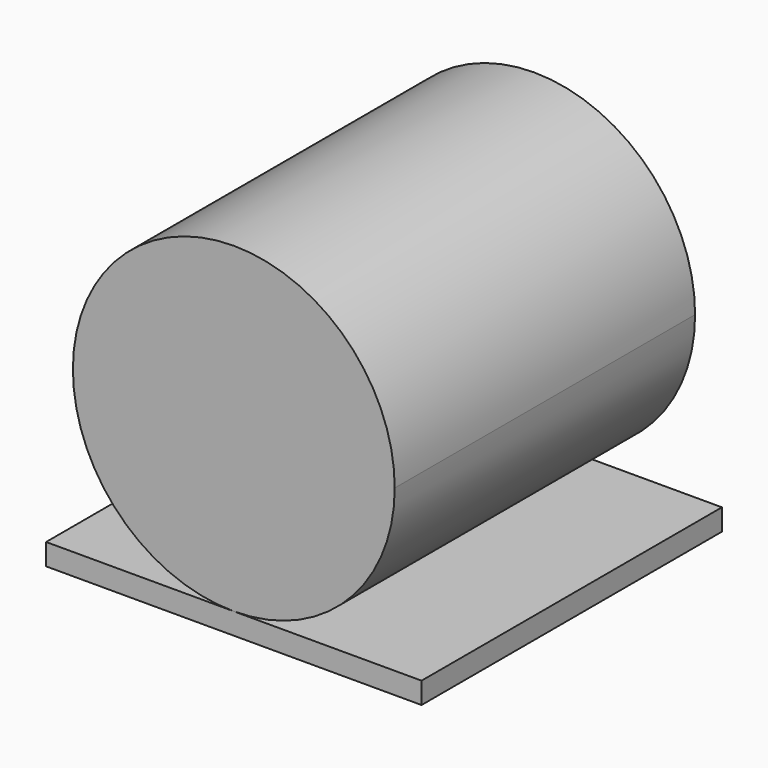
from build123d import *

# Parameters (mm, degrees)
F1_DEPTH = 88.9


# Not quite as in the source:
# - a feature names something its author has since deleted; it is built from what else it names


with BuildPart() as f1:
    # F0 (on Front) → F1 (new body)
    with BuildSketch(Plane.XZ):
        with BuildLine():
            ThreePointArc((-1.019e-07, -45.8680424225), (26.9407683272, -34.7088108218), (38.1, -7.7680424225))
            ThreePointArc((38.1, -7.7680424225), (-26.9407683272, 19.1727259767), (-1.019e-07, -45.8680424225))
        make_face()
    extrude(amount=F1_DEPTH)


with BuildPart() as f1b:
    # F0 (on Front) → F1, piece 2 (new body)
    with BuildSketch(Plane.XZ):
        Polygon((44.45, -45.8680424225), (-1.019e-07, -45.8680424225), (-44.45, -45.8680424225), (-44.45, -50.9480424225), (44.45, -50.9480424225), align=None)
    extrude(amount=F1_DEPTH)


solid = Compound([f1.part, f1b.part])
